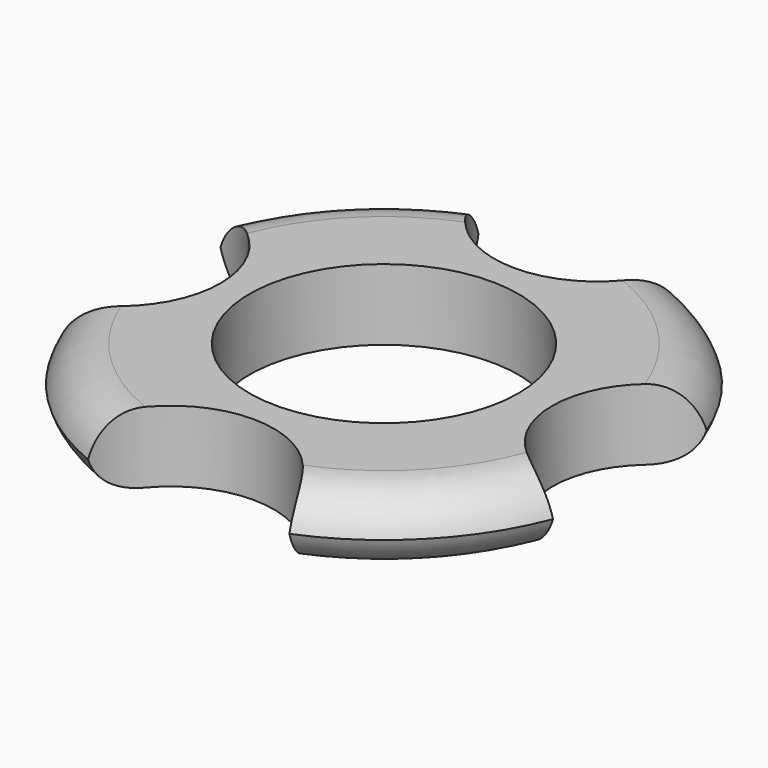
from build123d import *

# Parameters (mm, degrees)
F0_R         = 26.25
F1_DEPTH     = 7
F2_R         = 13.25
F3_DEPTH     = 25.4
F4_R         = 10.16
F4_R_2       = 9.6723514766
F5_DEPTH     = 25.4
F6_T2_ANGLE  = 101.8963155292
F6_T4_ANGLE  = 100.8121389037
F6_T6_ANGLE  = 100.8121389037
F6_T8_ANGLE  = 100.8121389037
F6_T10_ANGLE = 100.8121389037
F6_T12_ANGLE = 101.8963155292
F6_T14_ANGLE = 101.8963155292
F6_T16_ANGLE = 101.8963155292


# Not quite as in the source:
# - a fillet or chamfer that OpenCascade refuses, or shapes differently, is made with other operations: its cross-section is extruded or revolved along the edge and cut away or added


with BuildPart() as f1:
    # F0 (on Top) → F1 (new body)
    with BuildSketch(Plane.XY):
        Circle(F0_R)
    extrude(amount=F1_DEPTH)

    # F2 (on face) → F3 (cut)
    with BuildSketch(Plane.XY.offset(7)):
        Circle(F2_R)
    extrude(amount=-F3_DEPTH, mode=Mode.SUBTRACT)

    # F4 (on face) → F5 (cut)
    with BuildSketch(Plane.XY.offset(7)):
        with Locations((0, -26.25)):
            Circle(F4_R)
        with Locations((-26.25, 0)):
            Circle(F4_R)
        with Locations((0, 26.25)):
            Circle(F4_R)
        with Locations((26.25, 0)):
            Circle(F4_R_2)
    extrude(amount=-F5_DEPTH, mode=Mode.SUBTRACT)

    # F6: fillet of radius 5.08 on 8 edges, made by hand

    # F6_s1 → F6_t2 (revolve, cut)
    with BuildSketch(Plane(origin=(0, 0, 0), x_dir=(0, 0, 1), z_dir=(-0.995551765, 0.0942161515, 0))):
        with BuildLine():
            ThreePointArc((5.08, -26.25), (1.4878975516, -24.7621024484), (0, -21.17))
            Line((0, -21.17), (0, -26.25))
            Line((0, -26.25), (5.08, -26.25))
        make_face()
    revolve(axis=Axis((0, 0, 0), (0, 0, 1)), revolution_arc=F6_T2_ANGLE, mode=Mode.SUBTRACT)

    # F6_s3 → F6_t4 (revolve, cut)
    with BuildSketch(Plane(origin=(0, 0, 0), x_dir=(0, 0, 1), z_dir=(0.0942137746, 0.9955519899, 0))):
        with BuildLine():
            ThreePointArc((5.08, -26.25), (1.4878975516, -24.7621024484), (0, -21.17))
            Line((0, -21.17), (0, -26.25))
            Line((0, -26.25), (5.08, -26.25))
        make_face()
    revolve(axis=Axis((0, 0, 0), (0, 0, 1)), revolution_arc=F6_T4_ANGLE, mode=Mode.SUBTRACT)

    # F6_s5 → F6_t6 (revolve, cut)
    with BuildSketch(Plane(origin=(0, 0, 0), x_dir=(0, 0, 1), z_dir=(0.9955519899, -0.0942137746, 0))):
        with BuildLine():
            ThreePointArc((5.08, -26.25), (1.4878975516, -24.7621024484), (0, -21.17))
            Line((0, -21.17), (0, -26.25))
            Line((0, -26.25), (5.08, -26.25))
        make_face()
    revolve(axis=Axis((0, 0, 0), (0, 0, 1)), revolution_arc=F6_T6_ANGLE, mode=Mode.SUBTRACT)

    # F6_s7 → F6_t8 (revolve, cut)
    with BuildSketch(Plane(origin=(0, 0, 0), x_dir=(0, 0, 1), z_dir=(0.9955519899, -0.0942137746, 0))):
        with BuildLine():
            ThreePointArc((1.92, -26.25), (5.5121024484, -24.7621024484), (7, -21.17))
            Line((7, -21.17), (7, -26.25))
            Line((7, -26.25), (1.92, -26.25))
        make_face()
    revolve(axis=Axis((0, 0, 7), (0, 0, 1)), revolution_arc=F6_T8_ANGLE, mode=Mode.SUBTRACT)

    # F6_s9 → F6_t10 (revolve, cut)
    with BuildSketch(Plane(origin=(0, 0, 0), x_dir=(0, 0, 1), z_dir=(0.0942137746, 0.9955519899, 0))):
        with BuildLine():
            ThreePointArc((1.92, -26.25), (5.5121024484, -24.7621024484), (7, -21.17))
            Line((7, -21.17), (7, -26.25))
            Line((7, -26.25), (1.92, -26.25))
        make_face()
    revolve(axis=Axis((0, 0, 7), (0, 0, 1)), revolution_arc=F6_T10_ANGLE, mode=Mode.SUBTRACT)

    # F6_s11 → F6_t12 (revolve, cut)
    with BuildSketch(Plane(origin=(0, 0, 0), x_dir=(0, 0, 1), z_dir=(-0.995551765, 0.0942161515, 0))):
        with BuildLine():
            ThreePointArc((1.92, -26.25), (5.5121024484, -24.7621024484), (7, -21.17))
            Line((7, -21.17), (7, -26.25))
            Line((7, -26.25), (1.92, -26.25))
        make_face()
    revolve(axis=Axis((0, 0, 7), (0, 0, 1)), revolution_arc=F6_T12_ANGLE, mode=Mode.SUBTRACT)

    # F6_s13 → F6_t14 (revolve, cut)
    with BuildSketch(Plane(origin=(0, 0, 0), x_dir=(0, 0, 1), z_dir=(-0.1130316961, -0.9935913826, 0))):
        with BuildLine():
            ThreePointArc((1.92, -26.25), (5.5121024484, -24.7621024484), (7, -21.17))
            Line((7, -21.17), (7, -26.25))
            Line((7, -26.25), (1.92, -26.25))
        make_face()
    revolve(axis=Axis((0, 0, 7), (0, 0, 1)), revolution_arc=F6_T14_ANGLE, mode=Mode.SUBTRACT)

    # F6_s15 → F6_t16 (revolve, cut)
    with BuildSketch(Plane(origin=(0, 0, 0), x_dir=(0, 0, 1), z_dir=(-0.1130316961, -0.9935913826, 0))):
        with BuildLine():
            ThreePointArc((5.08, -26.25), (1.4878975516, -24.7621024484), (0, -21.17))
            Line((0, -21.17), (0, -26.25))
            Line((0, -26.25), (5.08, -26.25))
        make_face()
    revolve(axis=Axis((0, 0, 0), (0, 0, 1)), revolution_arc=F6_T16_ANGLE, mode=Mode.SUBTRACT)


solid = f1.part
